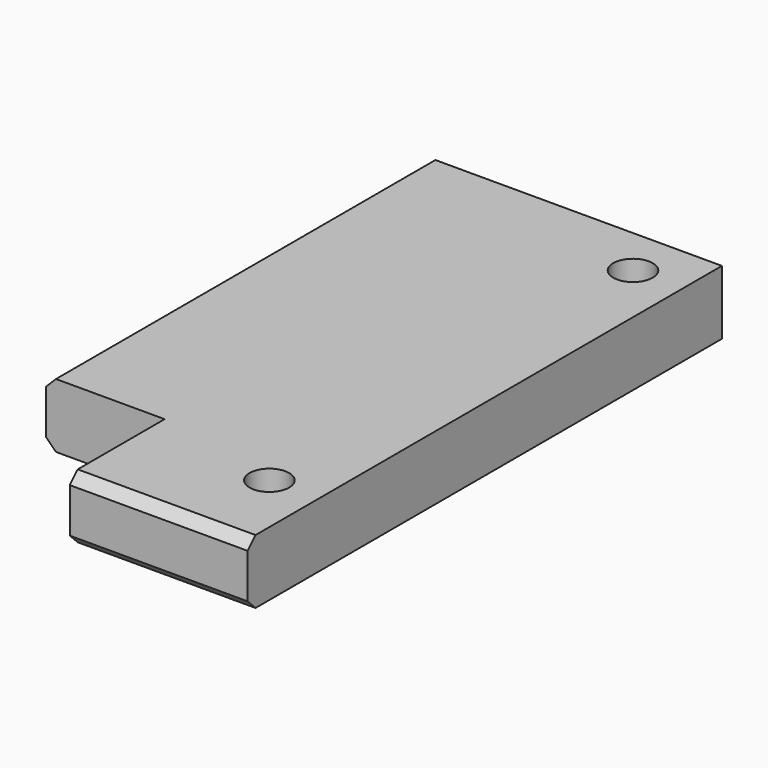
from build123d import *

# Parameters (mm, degrees)
F0_R     = 2
F1_DEPTH = 6.5
F2_SIZE  = 1


# Not quite as in the source:
# - a feature names something its author has since deleted; it is built from what else it names


with BuildPart() as f1:
    # F0 (on Top) → F1 (new body)
    with BuildSketch(Plane.XY):
        Polygon((12, 12), (12, 0), (30, 0), (30, 60), (0, 60), (0, 12), align=None)
        with Locations((25, 9)):
            Circle(F0_R, mode=Mode.SUBTRACT)
        with Locations((25, 55)):
            Circle(F0_R, mode=Mode.SUBTRACT)
    extrude(amount=F1_DEPTH)

    # F2
    f2_edges = [f1.edges().sort_by_distance(p)[0] for p in [
        (21, 0, 0),
        (21, 0, 6.5),
        (0, 36, 0),
        (0, 36, 6.5),
    ]]
    chamfer(f2_edges, length=F2_SIZE)


solid = f1.part
